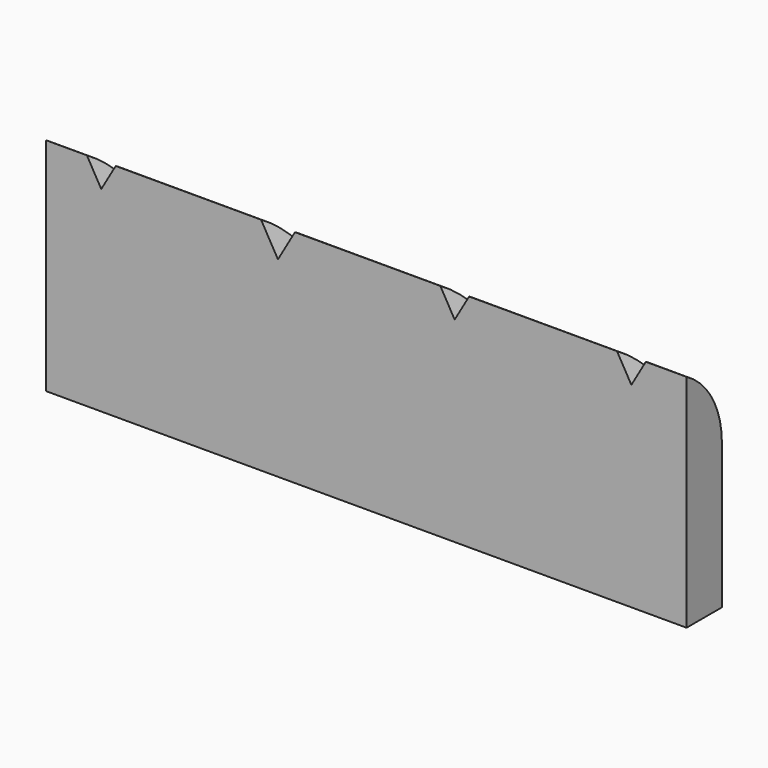
from build123d import *

# Parameters (mm, degrees)
F0_W        = 36.83
F0_H        = 2.54
F1_DEPTH    = 12.7
F3_T1_DEPTH = 58.8270452561
F4_DEPTH    = 25.4


# Not quite as in the source:
# - a fillet or chamfer that OpenCascade refuses, or shapes differently, is made with other operations: its cross-section is extruded or revolved along the edge and cut away or added


with BuildPart() as f1:
    # F0 (on Top) → F1 (new body)
    with BuildSketch(Plane.XY):
        with Locations((-0.635, 1.27)):
            Rectangle(F0_W, F0_H)
    extrude(amount=F1_DEPTH)

    # F3: fillet of radius 5.08 on 1 edges, made by hand

    # F3_s2 → F3_t1 (cut)
    with BuildSketch(Plane.YZ.offset(-30.0485226281)):
        with BuildLine():
            ThreePointArc((2.54, 8.3005909488), (1.8594090512, 10.8405909488), (0, 12.7))
            Line((0, 12.7), (2.54, 12.7))
            Line((2.54, 12.7), (2.54, 8.3005909488))
        make_face()
    extrude(amount=F3_T1_DEPTH, mode=Mode.SUBTRACT)

    # F2 (on face) → F4 (cut)
    with BuildSketch(Plane.XZ):
        Polygon((-15.875, 11.2622954744), (-15.0449409051, 12.7), (-16.7050590949, 12.7), align=None)
        Polygon((-4.7382939367, 12.7), (-6.6917060633, 12.7), (-5.715, 11.0082954744), align=None)
        Polygon((5.2750590949, 12.7), (3.6149409051, 12.7), (4.445, 11.2622954744), align=None)
        Polygon((15.4350590949, 12.7), (13.7749409051, 12.7), (14.605, 11.2622954744), align=None)
    extrude(amount=-F4_DEPTH, mode=Mode.SUBTRACT)


solid = f1.part
